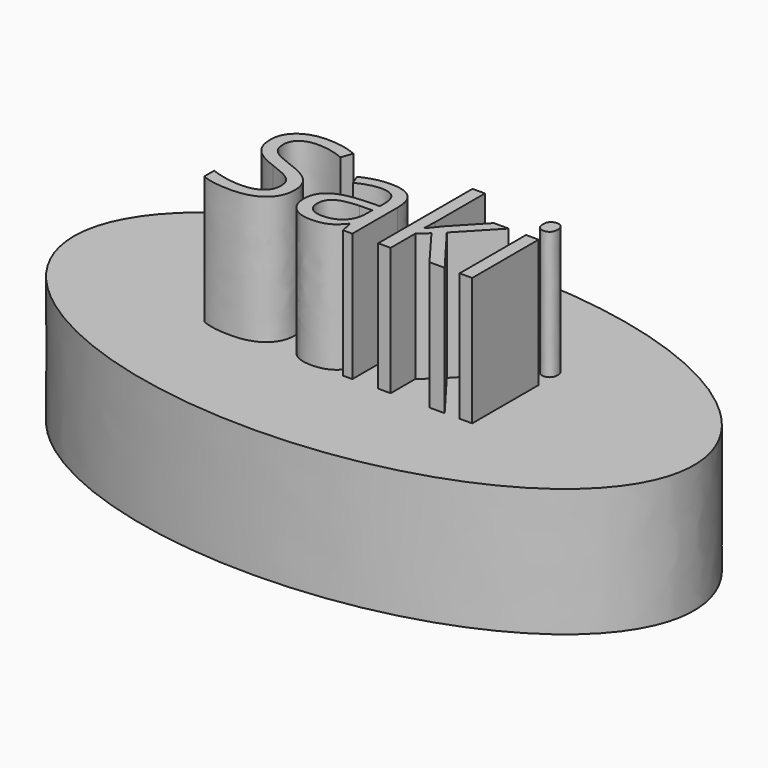
from build123d import *

# Parameters (mm, degrees)
F1_DEPTH     = 25.4
F2_TEXT_SIZE = 30.7719158526
F3_DEPTH     = 25.4


# Not quite as in the source:
# - Text() gives the source's letters only with a copy of the font that has no kerning and outlines rounded to 1/6400 em; it was checked with that copy


with BuildPart() as f1:
    # F0 (on Top) → F1 (new body)
    with BuildSketch(Plane.XY):
        with BuildLine():
            add(Edge.make_bspline(
                [(-61.5113675594, 0), (-61.5113675594, -57.7236308833), (30.7556837797, -28.8618154417), (123.0227351189, 0), (30.7556837797, 28.8618154417), (-61.5113675594, 57.7236308833), (-61.5113675594, 0)],
                knots=[0, 0, 0, 2.0943951024, 2.0943951024, 4.1887902048, 4.1887902048, 6.2831853072, 6.2831853072, 6.2831853072], degree=2, weights=[1, 0.5, 1, 0.5, 1, 0.5, 1]))
        make_face()
    extrude(amount=F1_DEPTH)

    # F2 (on face) → F3 (join)
    with BuildSketch(Plane.XY.offset(25.4)):
        with Locations((-29.3785855174, -10.5171082541)):
            Text('Saki', F2_TEXT_SIZE, font='Open Sans', text_align=(TextAlign.LEFT, TextAlign.BOTTOM))
    extrude(amount=F3_DEPTH)


solid = f1.part
